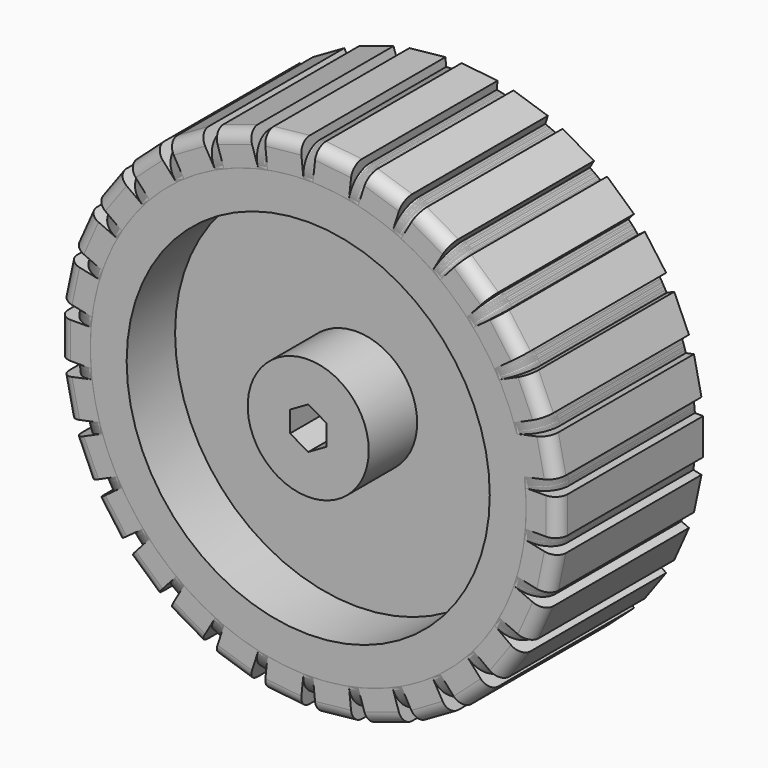
from build123d import *

# Parameters (mm, degrees)
F1_DEPTH        = 15
F1_COPIES_COUNT = 30
F2_R            = 2
F2_2_R          = 2
F2_3_R          = 2
F2_4_R          = 2
F2_5_R          = 2
F2_6_R          = 2
F2_7_R          = 2
F2_8_R          = 2
F2_9_R          = 2
F2_10_R         = 2
F2_11_R         = 2
F2_12_R         = 2
F2_13_R         = 2
F2_14_R         = 2
F2_15_R         = 2
F2_16_R         = 2
F2_17_R         = 2
F2_18_R         = 2
F2_19_R         = 2
F2_20_R         = 2
F2_21_R         = 2
F2_22_R         = 2
F2_23_R         = 2
F2_24_R         = 2
F2_25_R         = 2
F2_26_R         = 2
F2_27_R         = 2
F2_28_R         = 2
F2_29_R         = 2
F2_30_R         = 2
F3_R            = 15
F3_R_2          = 5
F4_DEPTH        = 5
F6_R            = 1
F6_2_R          = 1
F6_3_R          = 1
F6_4_R          = 1
F6_5_R          = 1
F6_6_R          = 1
F6_7_R          = 1
F6_8_R          = 1
F6_9_R          = 1
F6_10_R         = 1
F6_11_R         = 1
F6_12_R         = 1
F6_13_R         = 1
F6_14_R         = 1
F6_15_R         = 1
F6_16_R         = 1
F6_17_R         = 1
F6_18_R         = 1
F6_19_R         = 1
F6_20_R         = 1
F6_21_R         = 1
F6_22_R         = 1
F6_23_R         = 1
F6_24_R         = 1
F6_25_R         = 1
F6_26_R         = 1
F6_27_R         = 1
F6_28_R         = 1
F6_29_R         = 1
F6_30_R         = 1
F8_DEPTH        = 25


# Not quite as in the source:
# - a pattern or mirror of a feature is missing from the dataset's text; its kind, count and spacing are read off the source's solid


with BuildPart() as f1:
    # F0 (on Front) → F1 (new body)
    with BuildSketch(Plane.XZ):
        with BuildLine():
            ThreePointArc((19.944003923, -1.4955626102), (19.985996078, -0.7483052655), (20, 0))
            ThreePointArc((20, 0), (19.985996078, 0.7483052655), (19.944003923, 1.4955626102))
            Line((19.944003923, 1.4955626102), (19.3711882085, 1.4955626102))
            Line((19.3711882085, 1.4955626102), (19.3711882085, -1.4955626102))
            Line((19.3711882085, -1.4955626102), (19.944003923, -1.4955626102))
        make_face()
        with BuildLine():
            ThreePointArc((19.944003923, 1.4955626102), (19.985996078, 0.7483052655), (20, 0))
            ThreePointArc((20, 0), (19.985996078, -0.7483052655), (19.944003923, -1.4955626102))
            Line((19.944003923, -1.4955626102), (20.6288117915, -1.4955626102))
            Line((20.6288117915, -1.4955626102), (20.6288117915, 1.4955626102))
            Line((20.6288117915, 1.4955626102), (19.944003923, 1.4955626102))
        make_face()
        with BuildLine():
            Line((19.3711882085, 1.4955626102), (19.944003923, 1.4955626102))
            ThreePointArc((19.944003923, 1.4955626102), (-20, 0), (19.944003923, -1.4955626102))
            Line((19.944003923, -1.4955626102), (19.3711882085, -1.4955626102))
            Line((19.3711882085, -1.4955626102), (19.3711882085, 1.4955626102))
        make_face()
    extrude(amount=F1_DEPTH)


with BuildPart() as f1_copies_1:
    # F1_copies: instance of F1
    add(f1.part.rotate(Axis((0, 0, 0), (0, 1, 0)), 1 * 360 / F1_COPIES_COUNT))

    # F2#2
    f2_2_edges = [f1_copies_1.edges().sort_by_distance(p)[0] for p in [
        (-19.562952, -15, 4.158234),
    ]]
    fillet(f2_2_edges, radius=F2_2_R)


with BuildPart() as f1_copies_2:
    # F1_copies: instance of F1
    add(f1.part.rotate(Axis((0, 0, 0), (0, 1, 0)), 2 * 360 / F1_COPIES_COUNT))

    # F2#3
    f2_3_edges = [f1_copies_2.edges().sort_by_distance(p)[0] for p in [
        (-18.270909, -15, 8.134733),
    ]]
    fillet(f2_3_edges, radius=F2_3_R)


with BuildPart() as f1_copies_3:
    # F1_copies: instance of F1
    add(f1.part.rotate(Axis((0, 0, 0), (0, 1, 0)), 3 * 360 / F1_COPIES_COUNT))

    # F2#4
    f2_4_edges = [f1_copies_3.edges().sort_by_distance(p)[0] for p in [
        (-16.18034, -15, 11.755705),
    ]]
    fillet(f2_4_edges, radius=F2_4_R)


with BuildPart() as f1_copies_4:
    # F1_copies: instance of F1
    add(f1.part.rotate(Axis((0, 0, 0), (0, 1, 0)), 4 * 360 / F1_COPIES_COUNT))

    # F2#5
    f2_5_edges = [f1_copies_4.edges().sort_by_distance(p)[0] for p in [
        (-13.382612, -15, 14.862897),
    ]]
    fillet(f2_5_edges, radius=F2_5_R)


with BuildPart() as f1_copies_5:
    # F1_copies: instance of F1
    add(f1.part.rotate(Axis((0, 0, 0), (0, 1, 0)), 5 * 360 / F1_COPIES_COUNT))

    # F2#6
    f2_6_edges = [f1_copies_5.edges().sort_by_distance(p)[0] for p in [
        (-10, -15, 17.320508),
    ]]
    fillet(f2_6_edges, radius=F2_6_R)


with BuildPart() as f1_copies_6:
    # F1_copies: instance of F1
    add(f1.part.rotate(Axis((0, 0, 0), (0, 1, 0)), 6 * 360 / F1_COPIES_COUNT))

    # F2#7
    f2_7_edges = [f1_copies_6.edges().sort_by_distance(p)[0] for p in [
        (-6.18034, -15, 19.02113),
    ]]
    fillet(f2_7_edges, radius=F2_7_R)


with BuildPart() as f1_copies_7:
    # F1_copies: instance of F1
    add(f1.part.rotate(Axis((0, 0, 0), (0, 1, 0)), 7 * 360 / F1_COPIES_COUNT))

    # F2#8
    f2_8_edges = [f1_copies_7.edges().sort_by_distance(p)[0] for p in [
        (-2.090569, -15, 19.890438),
    ]]
    fillet(f2_8_edges, radius=F2_8_R)


with BuildPart() as f1_copies_8:
    # F1_copies: instance of F1
    add(f1.part.rotate(Axis((0, 0, 0), (0, 1, 0)), 8 * 360 / F1_COPIES_COUNT))

    # F2#9
    f2_9_edges = [f1_copies_8.edges().sort_by_distance(p)[0] for p in [
        (2.090569, -15, 19.890438),
    ]]
    fillet(f2_9_edges, radius=F2_9_R)


with BuildPart() as f1_copies_9:
    # F1_copies: instance of F1
    add(f1.part.rotate(Axis((0, 0, 0), (0, 1, 0)), 9 * 360 / F1_COPIES_COUNT))

    # F2#10
    f2_10_edges = [f1_copies_9.edges().sort_by_distance(p)[0] for p in [
        (6.18034, -15, 19.02113),
    ]]
    fillet(f2_10_edges, radius=F2_10_R)


with BuildPart() as f1_copies_10:
    # F1_copies: instance of F1
    add(f1.part.rotate(Axis((0, 0, 0), (0, 1, 0)), 10 * 360 / F1_COPIES_COUNT))

    # F2#11
    f2_11_edges = [f1_copies_10.edges().sort_by_distance(p)[0] for p in [
        (10, -15, 17.320508),
    ]]
    fillet(f2_11_edges, radius=F2_11_R)


with BuildPart() as f1_copies_11:
    # F1_copies: instance of F1
    add(f1.part.rotate(Axis((0, 0, 0), (0, 1, 0)), 11 * 360 / F1_COPIES_COUNT))

    # F2#12
    f2_12_edges = [f1_copies_11.edges().sort_by_distance(p)[0] for p in [
        (13.382612, -15, 14.862897),
    ]]
    fillet(f2_12_edges, radius=F2_12_R)


with BuildPart() as f1_copies_12:
    # F1_copies: instance of F1
    add(f1.part.rotate(Axis((0, 0, 0), (0, 1, 0)), 12 * 360 / F1_COPIES_COUNT))

    # F2#13
    f2_13_edges = [f1_copies_12.edges().sort_by_distance(p)[0] for p in [
        (16.18034, -15, 11.755705),
    ]]
    fillet(f2_13_edges, radius=F2_13_R)


with BuildPart() as f1_copies_13:
    # F1_copies: instance of F1
    add(f1.part.rotate(Axis((0, 0, 0), (0, 1, 0)), 13 * 360 / F1_COPIES_COUNT))

    # F2#14
    f2_14_edges = [f1_copies_13.edges().sort_by_distance(p)[0] for p in [
        (18.270909, -15, 8.134733),
    ]]
    fillet(f2_14_edges, radius=F2_14_R)


with BuildPart() as f1_copies_14:
    # F1_copies: instance of F1
    add(f1.part.rotate(Axis((0, 0, 0), (0, 1, 0)), 14 * 360 / F1_COPIES_COUNT))

    # F2#15
    f2_15_edges = [f1_copies_14.edges().sort_by_distance(p)[0] for p in [
        (19.562952, -15, 4.158234),
    ]]
    fillet(f2_15_edges, radius=F2_15_R)


with BuildPart() as f1_copies_15:
    # F1_copies: instance of F1
    add(f1.part.rotate(Axis((0, 0, 0), (0, 1, 0)), 15 * 360 / F1_COPIES_COUNT))

    # F2#16
    f2_16_edges = [f1_copies_15.edges().sort_by_distance(p)[0] for p in [
        (20, -15, 0),
    ]]
    fillet(f2_16_edges, radius=F2_16_R)


with BuildPart() as f1_copies_16:
    # F1_copies: instance of F1
    add(f1.part.rotate(Axis((0, 0, 0), (0, 1, 0)), 16 * 360 / F1_COPIES_COUNT))

    # F2#17
    f2_17_edges = [f1_copies_16.edges().sort_by_distance(p)[0] for p in [
        (19.562952, -15, -4.158234),
    ]]
    fillet(f2_17_edges, radius=F2_17_R)


with BuildPart() as f1_copies_17:
    # F1_copies: instance of F1
    add(f1.part.rotate(Axis((0, 0, 0), (0, 1, 0)), 17 * 360 / F1_COPIES_COUNT))

    # F2#18
    f2_18_edges = [f1_copies_17.edges().sort_by_distance(p)[0] for p in [
        (18.270909, -15, -8.134733),
    ]]
    fillet(f2_18_edges, radius=F2_18_R)


with BuildPart() as f1_copies_18:
    # F1_copies: instance of F1
    add(f1.part.rotate(Axis((0, 0, 0), (0, 1, 0)), 18 * 360 / F1_COPIES_COUNT))

    # F2#19
    f2_19_edges = [f1_copies_18.edges().sort_by_distance(p)[0] for p in [
        (16.18034, -15, -11.755705),
    ]]
    fillet(f2_19_edges, radius=F2_19_R)


with BuildPart() as f1_copies_19:
    # F1_copies: instance of F1
    add(f1.part.rotate(Axis((0, 0, 0), (0, 1, 0)), 19 * 360 / F1_COPIES_COUNT))

    # F2#20
    f2_20_edges = [f1_copies_19.edges().sort_by_distance(p)[0] for p in [
        (13.382612, -15, -14.862897),
    ]]
    fillet(f2_20_edges, radius=F2_20_R)


with BuildPart() as f1_copies_20:
    # F1_copies: instance of F1
    add(f1.part.rotate(Axis((0, 0, 0), (0, 1, 0)), 20 * 360 / F1_COPIES_COUNT))

    # F2#21
    f2_21_edges = [f1_copies_20.edges().sort_by_distance(p)[0] for p in [
        (10, -15, -17.320508),
    ]]
    fillet(f2_21_edges, radius=F2_21_R)


with BuildPart() as f1_copies_21:
    # F1_copies: instance of F1
    add(f1.part.rotate(Axis((0, 0, 0), (0, 1, 0)), 21 * 360 / F1_COPIES_COUNT))

    # F2#22
    f2_22_edges = [f1_copies_21.edges().sort_by_distance(p)[0] for p in [
        (6.18034, -15, -19.02113),
    ]]
    fillet(f2_22_edges, radius=F2_22_R)


with BuildPart() as f1_copies_22:
    # F1_copies: instance of F1
    add(f1.part.rotate(Axis((0, 0, 0), (0, 1, 0)), 22 * 360 / F1_COPIES_COUNT))

    # F2#23
    f2_23_edges = [f1_copies_22.edges().sort_by_distance(p)[0] for p in [
        (2.090569, -15, -19.890438),
    ]]
    fillet(f2_23_edges, radius=F2_23_R)


with BuildPart() as f1_copies_23:
    # F1_copies: instance of F1
    add(f1.part.rotate(Axis((0, 0, 0), (0, 1, 0)), 23 * 360 / F1_COPIES_COUNT))

    # F2#24
    f2_24_edges = [f1_copies_23.edges().sort_by_distance(p)[0] for p in [
        (-2.090569, -15, -19.890438),
    ]]
    fillet(f2_24_edges, radius=F2_24_R)


with BuildPart() as f1_copies_24:
    # F1_copies: instance of F1
    add(f1.part.rotate(Axis((0, 0, 0), (0, 1, 0)), 24 * 360 / F1_COPIES_COUNT))

    # F2#25
    f2_25_edges = [f1_copies_24.edges().sort_by_distance(p)[0] for p in [
        (-6.18034, -15, -19.02113),
    ]]
    fillet(f2_25_edges, radius=F2_25_R)


with BuildPart() as f1_copies_25:
    # F1_copies: instance of F1
    add(f1.part.rotate(Axis((0, 0, 0), (0, 1, 0)), 25 * 360 / F1_COPIES_COUNT))

    # F2#26
    f2_26_edges = [f1_copies_25.edges().sort_by_distance(p)[0] for p in [
        (-10, -15, -17.320508),
    ]]
    fillet(f2_26_edges, radius=F2_26_R)


with BuildPart() as f1_copies_26:
    # F1_copies: instance of F1
    add(f1.part.rotate(Axis((0, 0, 0), (0, 1, 0)), 26 * 360 / F1_COPIES_COUNT))

    # F2#27
    f2_27_edges = [f1_copies_26.edges().sort_by_distance(p)[0] for p in [
        (-13.382612, -15, -14.862897),
    ]]
    fillet(f2_27_edges, radius=F2_27_R)


with BuildPart() as f1_copies_27:
    # F1_copies: instance of F1
    add(f1.part.rotate(Axis((0, 0, 0), (0, 1, 0)), 27 * 360 / F1_COPIES_COUNT))

    # F2#28
    f2_28_edges = [f1_copies_27.edges().sort_by_distance(p)[0] for p in [
        (-16.18034, -15, -11.755705),
    ]]
    fillet(f2_28_edges, radius=F2_28_R)


with BuildPart() as f1_copies_28:
    # F1_copies: instance of F1
    add(f1.part.rotate(Axis((0, 0, 0), (0, 1, 0)), 28 * 360 / F1_COPIES_COUNT))

    # F2#29
    f2_29_edges = [f1_copies_28.edges().sort_by_distance(p)[0] for p in [
        (-18.270909, -15, -8.134733),
    ]]
    fillet(f2_29_edges, radius=F2_29_R)


with BuildPart() as f1_copies_29:
    # F1_copies: instance of F1
    add(f1.part.rotate(Axis((0, 0, 0), (0, 1, 0)), 29 * 360 / F1_COPIES_COUNT))

    # F2#30
    f2_30_edges = [f1_copies_29.edges().sort_by_distance(p)[0] for p in [
        (-19.562952, -15, -4.158234),
    ]]
    fillet(f2_30_edges, radius=F2_30_R)


with BuildPart() as f1_1:
    add(f1.part)

    # F2
    f2_edges = [f1_1.edges().sort_by_distance(p)[0] for p in [
        (-20, -15, 0),
    ]]
    fillet(f2_edges, radius=F2_R)


with BuildPart() as f4_tool:
    # F3 (on face) → F4 (new body)
    with BuildSketch(Plane.XZ.offset(15)):
        Circle(F3_R)
        Circle(F3_R_2, mode=Mode.SUBTRACT)
    extrude(amount=-F4_DEPTH)


with BuildPart() as f1_2:
    add(f1_1.part)

    # F4: cut by f4_tool
    add(f4_tool.part, mode=Mode.SUBTRACT)

    # F6
    f6_edges = [f1_2.edges().sort_by_distance(p)[0] for p in [
        (20.628812, -15, 0),
    ]]
    fillet(f6_edges, radius=F6_R)


with BuildPart() as f1_copies_1_1:
    add(f1_copies_1.part)

    # F4: cut by f4_tool
    add(f4_tool.part, mode=Mode.SUBTRACT)

    # F6#2
    f6_2_edges = [f1_copies_1_1.edges().sort_by_distance(p)[0] for p in [
        (20.178023, -15, -4.288971),
    ]]
    fillet(f6_2_edges, radius=F6_2_R)


with BuildPart() as f1_copies_2_1:
    add(f1_copies_2.part)

    # F4: cut by f4_tool
    add(f4_tool.part, mode=Mode.SUBTRACT)

    # F6#3
    f6_3_edges = [f1_copies_2_1.edges().sort_by_distance(p)[0] for p in [
        (18.845357, -15, -8.390494),
    ]]
    fillet(f6_3_edges, radius=F6_3_R)


with BuildPart() as f1_copies_3_1:
    add(f1_copies_3.part)

    # F4: cut by f4_tool
    add(f4_tool.part, mode=Mode.SUBTRACT)

    # F6#4
    f6_4_edges = [f1_copies_3_1.edges().sort_by_distance(p)[0] for p in [
        (16.689059, -15, -12.125311),
    ]]
    fillet(f6_4_edges, radius=F6_4_R)


with BuildPart() as f1_copies_4_1:
    add(f1_copies_4.part)

    # F4: cut by f4_tool
    add(f4_tool.part, mode=Mode.SUBTRACT)

    # F6#5
    f6_5_edges = [f1_copies_4_1.edges().sort_by_distance(p)[0] for p in [
        (13.803369, -15, -15.330195),
    ]]
    fillet(f6_5_edges, radius=F6_5_R)


with BuildPart() as f1_copies_5_1:
    add(f1_copies_5.part)

    # F4: cut by f4_tool
    add(f4_tool.part, mode=Mode.SUBTRACT)

    # F6#6
    f6_6_edges = [f1_copies_5_1.edges().sort_by_distance(p)[0] for p in [
        (10.314406, -15, -17.865075),
    ]]
    fillet(f6_6_edges, radius=F6_6_R)


with BuildPart() as f1_copies_6_1:
    add(f1_copies_6.part)

    # F4: cut by f4_tool
    add(f4_tool.part, mode=Mode.SUBTRACT)

    # F6#7
    f6_7_edges = [f1_copies_6_1.edges().sort_by_distance(p)[0] for p in [
        (6.374653, -15, -19.619166),
    ]]
    fillet(f6_7_edges, radius=F6_7_R)


with BuildPart() as f1_copies_7_1:
    add(f1_copies_7.part)

    # F4: cut by f4_tool
    add(f4_tool.part, mode=Mode.SUBTRACT)

    # F6#8
    f6_8_edges = [f1_copies_7_1.edges().sort_by_distance(p)[0] for p in [
        (2.156298, -15, -20.515805),
    ]]
    fillet(f6_8_edges, radius=F6_8_R)


with BuildPart() as f1_copies_8_1:
    add(f1_copies_8.part)

    # F4: cut by f4_tool
    add(f4_tool.part, mode=Mode.SUBTRACT)

    # F6#9
    f6_9_edges = [f1_copies_8_1.edges().sort_by_distance(p)[0] for p in [
        (-2.156298, -15, -20.515805),
    ]]
    fillet(f6_9_edges, radius=F6_9_R)


with BuildPart() as f1_copies_9_1:
    add(f1_copies_9.part)

    # F4: cut by f4_tool
    add(f4_tool.part, mode=Mode.SUBTRACT)

    # F6#10
    f6_10_edges = [f1_copies_9_1.edges().sort_by_distance(p)[0] for p in [
        (-6.374653, -15, -19.619166),
    ]]
    fillet(f6_10_edges, radius=F6_10_R)


with BuildPart() as f1_copies_10_1:
    add(f1_copies_10.part)

    # F4: cut by f4_tool
    add(f4_tool.part, mode=Mode.SUBTRACT)

    # F6#11
    f6_11_edges = [f1_copies_10_1.edges().sort_by_distance(p)[0] for p in [
        (-10.314406, -15, -17.865075),
    ]]
    fillet(f6_11_edges, radius=F6_11_R)


with BuildPart() as f1_copies_11_1:
    add(f1_copies_11.part)

    # F4: cut by f4_tool
    add(f4_tool.part, mode=Mode.SUBTRACT)

    # F6#12
    f6_12_edges = [f1_copies_11_1.edges().sort_by_distance(p)[0] for p in [
        (-13.803369, -15, -15.330195),
    ]]
    fillet(f6_12_edges, radius=F6_12_R)


with BuildPart() as f1_copies_12_1:
    add(f1_copies_12.part)

    # F4: cut by f4_tool
    add(f4_tool.part, mode=Mode.SUBTRACT)

    # F6#13
    f6_13_edges = [f1_copies_12_1.edges().sort_by_distance(p)[0] for p in [
        (-16.689059, -15, -12.125311),
    ]]
    fillet(f6_13_edges, radius=F6_13_R)


with BuildPart() as f1_copies_13_1:
    add(f1_copies_13.part)

    # F4: cut by f4_tool
    add(f4_tool.part, mode=Mode.SUBTRACT)

    # F6#14
    f6_14_edges = [f1_copies_13_1.edges().sort_by_distance(p)[0] for p in [
        (-18.845357, -15, -8.390494),
    ]]
    fillet(f6_14_edges, radius=F6_14_R)


with BuildPart() as f1_copies_14_1:
    add(f1_copies_14.part)

    # F4: cut by f4_tool
    add(f4_tool.part, mode=Mode.SUBTRACT)

    # F6#15
    f6_15_edges = [f1_copies_14_1.edges().sort_by_distance(p)[0] for p in [
        (-20.178023, -15, -4.288971),
    ]]
    fillet(f6_15_edges, radius=F6_15_R)


with BuildPart() as f1_copies_15_1:
    add(f1_copies_15.part)

    # F4: cut by f4_tool
    add(f4_tool.part, mode=Mode.SUBTRACT)

    # F6#16
    f6_16_edges = [f1_copies_15_1.edges().sort_by_distance(p)[0] for p in [
        (-20.628812, -15, 0),
    ]]
    fillet(f6_16_edges, radius=F6_16_R)


with BuildPart() as f1_copies_16_1:
    add(f1_copies_16.part)

    # F4: cut by f4_tool
    add(f4_tool.part, mode=Mode.SUBTRACT)

    # F6#17
    f6_17_edges = [f1_copies_16_1.edges().sort_by_distance(p)[0] for p in [
        (-20.178023, -15, 4.288971),
    ]]
    fillet(f6_17_edges, radius=F6_17_R)


with BuildPart() as f1_copies_17_1:
    add(f1_copies_17.part)

    # F4: cut by f4_tool
    add(f4_tool.part, mode=Mode.SUBTRACT)

    # F6#18
    f6_18_edges = [f1_copies_17_1.edges().sort_by_distance(p)[0] for p in [
        (-18.845357, -15, 8.390494),
    ]]
    fillet(f6_18_edges, radius=F6_18_R)


with BuildPart() as f1_copies_18_1:
    add(f1_copies_18.part)

    # F4: cut by f4_tool
    add(f4_tool.part, mode=Mode.SUBTRACT)

    # F6#19
    f6_19_edges = [f1_copies_18_1.edges().sort_by_distance(p)[0] for p in [
        (-16.689059, -15, 12.125311),
    ]]
    fillet(f6_19_edges, radius=F6_19_R)


with BuildPart() as f1_copies_19_1:
    add(f1_copies_19.part)

    # F4: cut by f4_tool
    add(f4_tool.part, mode=Mode.SUBTRACT)

    # F6#20
    f6_20_edges = [f1_copies_19_1.edges().sort_by_distance(p)[0] for p in [
        (-13.803369, -15, 15.330195),
    ]]
    fillet(f6_20_edges, radius=F6_20_R)


with BuildPart() as f1_copies_20_1:
    add(f1_copies_20.part)

    # F4: cut by f4_tool
    add(f4_tool.part, mode=Mode.SUBTRACT)

    # F6#21
    f6_21_edges = [f1_copies_20_1.edges().sort_by_distance(p)[0] for p in [
        (-10.314406, -15, 17.865075),
    ]]
    fillet(f6_21_edges, radius=F6_21_R)


with BuildPart() as f1_copies_21_1:
    add(f1_copies_21.part)

    # F4: cut by f4_tool
    add(f4_tool.part, mode=Mode.SUBTRACT)

    # F6#22
    f6_22_edges = [f1_copies_21_1.edges().sort_by_distance(p)[0] for p in [
        (-6.374653, -15, 19.619166),
    ]]
    fillet(f6_22_edges, radius=F6_22_R)


with BuildPart() as f1_copies_22_1:
    add(f1_copies_22.part)

    # F4: cut by f4_tool
    add(f4_tool.part, mode=Mode.SUBTRACT)

    # F6#23
    f6_23_edges = [f1_copies_22_1.edges().sort_by_distance(p)[0] for p in [
        (-2.156298, -15, 20.515805),
    ]]
    fillet(f6_23_edges, radius=F6_23_R)


with BuildPart() as f1_copies_23_1:
    add(f1_copies_23.part)

    # F4: cut by f4_tool
    add(f4_tool.part, mode=Mode.SUBTRACT)

    # F6#24
    f6_24_edges = [f1_copies_23_1.edges().sort_by_distance(p)[0] for p in [
        (2.156298, -15, 20.515805),
    ]]
    fillet(f6_24_edges, radius=F6_24_R)


with BuildPart() as f1_copies_24_1:
    add(f1_copies_24.part)

    # F4: cut by f4_tool
    add(f4_tool.part, mode=Mode.SUBTRACT)

    # F6#25
    f6_25_edges = [f1_copies_24_1.edges().sort_by_distance(p)[0] for p in [
        (6.374653, -15, 19.619166),
    ]]
    fillet(f6_25_edges, radius=F6_25_R)


with BuildPart() as f1_copies_25_1:
    add(f1_copies_25.part)

    # F4: cut by f4_tool
    add(f4_tool.part, mode=Mode.SUBTRACT)

    # F6#26
    f6_26_edges = [f1_copies_25_1.edges().sort_by_distance(p)[0] for p in [
        (10.314406, -15, 17.865075),
    ]]
    fillet(f6_26_edges, radius=F6_26_R)


with BuildPart() as f1_copies_26_1:
    add(f1_copies_26.part)

    # F4: cut by f4_tool
    add(f4_tool.part, mode=Mode.SUBTRACT)

    # F6#27
    f6_27_edges = [f1_copies_26_1.edges().sort_by_distance(p)[0] for p in [
        (13.803369, -15, 15.330195),
    ]]
    fillet(f6_27_edges, radius=F6_27_R)


with BuildPart() as f1_copies_27_1:
    add(f1_copies_27.part)

    # F4: cut by f4_tool
    add(f4_tool.part, mode=Mode.SUBTRACT)

    # F6#28
    f6_28_edges = [f1_copies_27_1.edges().sort_by_distance(p)[0] for p in [
        (16.689059, -15, 12.125311),
    ]]
    fillet(f6_28_edges, radius=F6_28_R)


with BuildPart() as f1_copies_28_1:
    add(f1_copies_28.part)

    # F4: cut by f4_tool
    add(f4_tool.part, mode=Mode.SUBTRACT)

    # F6#29
    f6_29_edges = [f1_copies_28_1.edges().sort_by_distance(p)[0] for p in [
        (18.845357, -15, 8.390494),
    ]]
    fillet(f6_29_edges, radius=F6_29_R)


with BuildPart() as f1_copies_29_1:
    add(f1_copies_29.part)

    # F4: cut by f4_tool
    add(f4_tool.part, mode=Mode.SUBTRACT)

    # F6#30
    f6_30_edges = [f1_copies_29_1.edges().sort_by_distance(p)[0] for p in [
        (20.178023, -15, 4.288971),
    ]]
    fillet(f6_30_edges, radius=F6_30_R)


with BuildPart() as f8_tool:
    # F7 (on face) → F8 (new body)
    with BuildSketch(Plane.XZ):
        Polygon((1.5, -0.8660254038), (1.5, 0.8660254038), (0, 1.7320508076), (-1.5, 0.8660254038), (-1.5, -0.8660254038), (0, -1.7320508076), align=None)
    extrude(amount=F8_DEPTH)


with BuildPart() as f1_3:
    add(f1_2.part)

    # F8: cut by f8_tool
    add(f8_tool.part, mode=Mode.SUBTRACT)


with BuildPart() as f1_copies_1_2:
    add(f1_copies_1_1.part)

    # F8: cut by f8_tool
    add(f8_tool.part, mode=Mode.SUBTRACT)


with BuildPart() as f1_copies_2_2:
    add(f1_copies_2_1.part)

    # F8: cut by f8_tool
    add(f8_tool.part, mode=Mode.SUBTRACT)


with BuildPart() as f1_copies_3_2:
    add(f1_copies_3_1.part)

    # F8: cut by f8_tool
    add(f8_tool.part, mode=Mode.SUBTRACT)


with BuildPart() as f1_copies_4_2:
    add(f1_copies_4_1.part)

    # F8: cut by f8_tool
    add(f8_tool.part, mode=Mode.SUBTRACT)


with BuildPart() as f1_copies_5_2:
    add(f1_copies_5_1.part)

    # F8: cut by f8_tool
    add(f8_tool.part, mode=Mode.SUBTRACT)


with BuildPart() as f1_copies_6_2:
    add(f1_copies_6_1.part)

    # F8: cut by f8_tool
    add(f8_tool.part, mode=Mode.SUBTRACT)


with BuildPart() as f1_copies_7_2:
    add(f1_copies_7_1.part)

    # F8: cut by f8_tool
    add(f8_tool.part, mode=Mode.SUBTRACT)


with BuildPart() as f1_copies_8_2:
    add(f1_copies_8_1.part)

    # F8: cut by f8_tool
    add(f8_tool.part, mode=Mode.SUBTRACT)


with BuildPart() as f1_copies_9_2:
    add(f1_copies_9_1.part)

    # F8: cut by f8_tool
    add(f8_tool.part, mode=Mode.SUBTRACT)


with BuildPart() as f1_copies_10_2:
    add(f1_copies_10_1.part)

    # F8: cut by f8_tool
    add(f8_tool.part, mode=Mode.SUBTRACT)


with BuildPart() as f1_copies_11_2:
    add(f1_copies_11_1.part)

    # F8: cut by f8_tool
    add(f8_tool.part, mode=Mode.SUBTRACT)


with BuildPart() as f1_copies_12_2:
    add(f1_copies_12_1.part)

    # F8: cut by f8_tool
    add(f8_tool.part, mode=Mode.SUBTRACT)


with BuildPart() as f1_copies_13_2:
    add(f1_copies_13_1.part)

    # F8: cut by f8_tool
    add(f8_tool.part, mode=Mode.SUBTRACT)


with BuildPart() as f1_copies_14_2:
    add(f1_copies_14_1.part)

    # F8: cut by f8_tool
    add(f8_tool.part, mode=Mode.SUBTRACT)


with BuildPart() as f1_copies_15_2:
    add(f1_copies_15_1.part)

    # F8: cut by f8_tool
    add(f8_tool.part, mode=Mode.SUBTRACT)


with BuildPart() as f1_copies_16_2:
    add(f1_copies_16_1.part)

    # F8: cut by f8_tool
    add(f8_tool.part, mode=Mode.SUBTRACT)


with BuildPart() as f1_copies_17_2:
    add(f1_copies_17_1.part)

    # F8: cut by f8_tool
    add(f8_tool.part, mode=Mode.SUBTRACT)


with BuildPart() as f1_copies_18_2:
    add(f1_copies_18_1.part)

    # F8: cut by f8_tool
    add(f8_tool.part, mode=Mode.SUBTRACT)


with BuildPart() as f1_copies_19_2:
    add(f1_copies_19_1.part)

    # F8: cut by f8_tool
    add(f8_tool.part, mode=Mode.SUBTRACT)


with BuildPart() as f1_copies_20_2:
    add(f1_copies_20_1.part)

    # F8: cut by f8_tool
    add(f8_tool.part, mode=Mode.SUBTRACT)


with BuildPart() as f1_copies_21_2:
    add(f1_copies_21_1.part)

    # F8: cut by f8_tool
    add(f8_tool.part, mode=Mode.SUBTRACT)


with BuildPart() as f1_copies_22_2:
    add(f1_copies_22_1.part)

    # F8: cut by f8_tool
    add(f8_tool.part, mode=Mode.SUBTRACT)


with BuildPart() as f1_copies_23_2:
    add(f1_copies_23_1.part)

    # F8: cut by f8_tool
    add(f8_tool.part, mode=Mode.SUBTRACT)


with BuildPart() as f1_copies_24_2:
    add(f1_copies_24_1.part)

    # F8: cut by f8_tool
    add(f8_tool.part, mode=Mode.SUBTRACT)


with BuildPart() as f1_copies_25_2:
    add(f1_copies_25_1.part)

    # F8: cut by f8_tool
    add(f8_tool.part, mode=Mode.SUBTRACT)


with BuildPart() as f1_copies_26_2:
    add(f1_copies_26_1.part)

    # F8: cut by f8_tool
    add(f8_tool.part, mode=Mode.SUBTRACT)


with BuildPart() as f1_copies_27_2:
    add(f1_copies_27_1.part)

    # F8: cut by f8_tool
    add(f8_tool.part, mode=Mode.SUBTRACT)


with BuildPart() as f1_copies_28_2:
    add(f1_copies_28_1.part)

    # F8: cut by f8_tool
    add(f8_tool.part, mode=Mode.SUBTRACT)


with BuildPart() as f1_copies_29_2:
    add(f1_copies_29_1.part)

    # F8: cut by f8_tool
    add(f8_tool.part, mode=Mode.SUBTRACT)


solid = Compound([f1_3.part, f1_copies_1_2.part, f1_copies_2_2.part, f1_copies_3_2.part, f1_copies_4_2.part, f1_copies_5_2.part, f1_copies_6_2.part, f1_copies_7_2.part, f1_copies_8_2.part, f1_copies_9_2.part, f1_copies_10_2.part, f1_copies_11_2.part, f1_copies_12_2.part, f1_copies_13_2.part, f1_copies_14_2.part, f1_copies_15_2.part, f1_copies_16_2.part, f1_copies_17_2.part, f1_copies_18_2.part, f1_copies_19_2.part, f1_copies_20_2.part, f1_copies_21_2.part, f1_copies_22_2.part, f1_copies_23_2.part, f1_copies_24_2.part, f1_copies_25_2.part, f1_copies_26_2.part, f1_copies_27_2.part, f1_copies_28_2.part, f1_copies_29_2.part])
